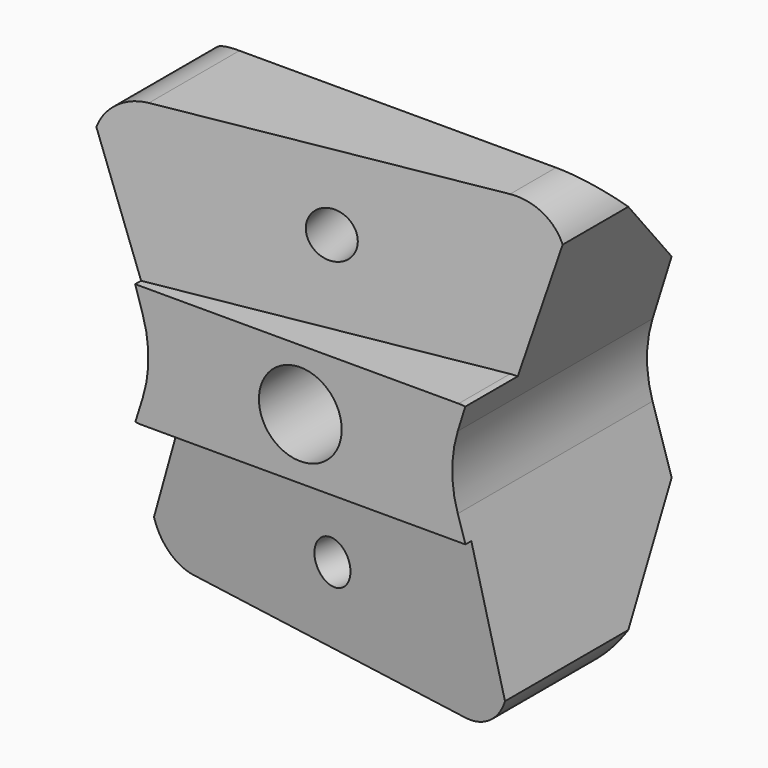
from build123d import *

# Parameters (mm, degrees)
F0_W      = 17
F0_H      = 18
F1_DEPTH  = 10
F2_R      = 1.7
F3_DEPTH  = 25
F5_DEPTH  = 6.5
F7_DEPTH  = 6.5
F8_SIZE   = 5
F9_R      = 2
F11_DEPTH = 25
F12_R     = 5
F13_R     = 0.95
F14_DEPTH = 25
F15_R     = 0.875
F16_DEPTH = 25
F17_R     = 0.95
F18_DEPTH = 25


# Not quite as in the source:
# - a feature names something its author has since deleted; it is built from what else it names


with BuildPart() as f1:
    # F0 (on Front) → F1 (new body)
    with BuildSketch(Plane.XZ):
        Rectangle(F0_W, F0_H)
    extrude(amount=F1_DEPTH)

    # F2 (on face) → F3 (cut)
    with BuildSketch(Plane.XZ.offset(10)):
        Circle(F2_R)
    extrude(amount=-F3_DEPTH, mode=Mode.SUBTRACT)

    # F4 (on face) → F5 (cut)
    with BuildSketch(Plane(origin=(0, 0, -9), x_dir=(1, 0, 0), z_dir=(0, 0, -1))):
        Polygon((8.5, 10), (-8.5, 10), (-8.5, 7.002441328), align=None)
    extrude(amount=-F5_DEPTH, mode=Mode.SUBTRACT)

    # F6 (on face) → F7 (cut)
    with BuildSketch(Plane.XY.offset(9)):
        Polygon((8.5, -7.002441328), (-8.5, -10), (8.5, -10), align=None)
    extrude(amount=-F7_DEPTH, mode=Mode.SUBTRACT)

    # F8
    f8_edges = [f1.edges().sort_by_distance(p)[0] for p in [
        (0, 0, 9),
        (0, 0, -9),
    ]]
    chamfer(f8_edges, length=F8_SIZE)

    # F9
    f9_edges = [f1.edges().sort_by_distance(p)[0] for p in [
        (8.5, -8.501221, 2.5),
        (-8.5, -8.501221, -2.5),
        (8.5, -7.5, -9),
        (-8.5, -6.001221, -9),
        (8.5, -6.001221, 9),
        (-8.5, -7.5, 9),
    ]]
    fillet(f9_edges, radius=F9_R)

    # F10 (on face) → F11 (cut)
    with BuildSketch(Plane.XZ.offset(10)):
        Polygon((-8.5, -8), (-6, 0), (-8.5, 8), align=None)
        Polygon((8.5, -8), (8.5, 8), (6, 0), align=None)
    extrude(amount=-F11_DEPTH, mode=Mode.SUBTRACT)

    # F12
    f12_edges = [f1.edges().sort_by_distance(p)[0] for p in [
        (-6, -5, 0),
        (6, -5, 0),
    ]]
    fillet(f12_edges, radius=F12_R)

    # F13 (on face) → F14 (cut)
    with BuildSketch(Plane(origin=(1.453794355, -8.2448774948, 0), x_dir=(0.984807753, 0.1736481777, 0), z_dir=(0.1736481777, -0.984807753, 0))):
        with Locations((-1.3918819604, 5.9)):
            Circle(F13_R)
    extrude(amount=-F14_DEPTH, mode=Mode.SUBTRACT)

    # F15 (on face) → F16 (cut)
    with BuildSketch(Plane(origin=(-1.453794355, -8.2448774948, 0), x_dir=(0.984807753, -0.1736481777, 0), z_dir=(-0.1736481777, -0.984807753, 0))):
        with Locations((1.6190158435, -5.9)):
            Circle(F15_R)
    extrude(amount=-F16_DEPTH, mode=Mode.SUBTRACT)

    # F17 (on Right) → F18 (cut)
    with BuildSketch(Plane.YZ):
        with Locations((-5, 0)):
            Circle(F17_R)
    extrude(amount=-F18_DEPTH, mode=Mode.SUBTRACT)


solid = f1.part
